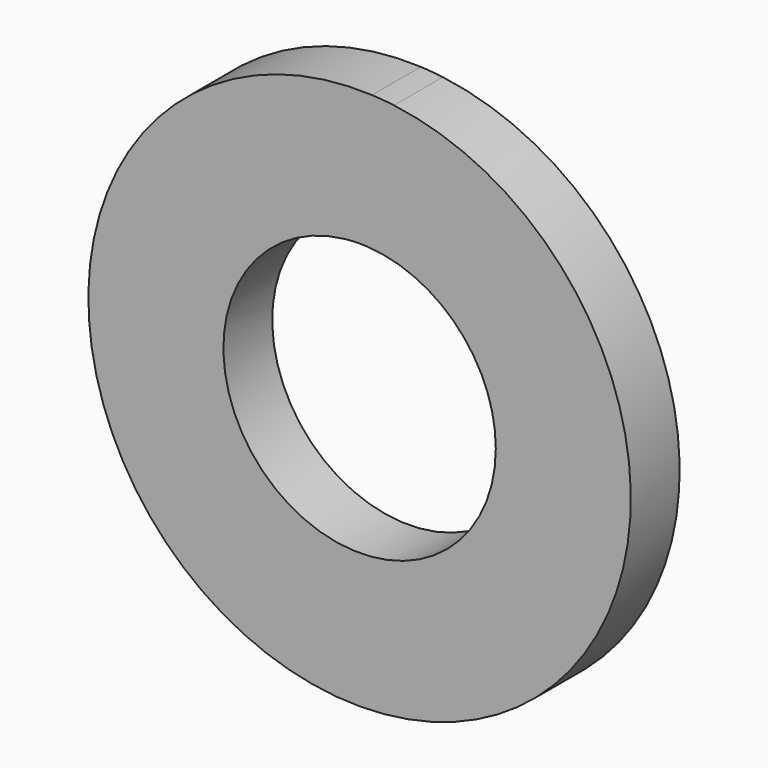
from build123d import *

# Parameters (mm, degrees)
F1_DEPTH = 15.494


# Not quite as in the source:
# - the program builds the solid bodies; features that only make, move or delete a surface that nothing else refers to are left out


with BuildPart() as f1:
    # F0 (on Front) → F1 (new body)
    with BuildSketch(Plane.XZ):
        with BuildLine():
            Line((1.9883703665, 34.5010177122), (8.7319990578, 68.2588214835))
            ThreePointArc((8.7319990578, 68.2588214835), (5.9467168888, 68.5576478309), (3.1515805748, 68.742869141))
            Line((3.1515805748, 68.742869141), (-3.7173636083, 34.3577509115))
            ThreePointArc((-3.7173636083, 34.3577509115), (-0.867459366, 34.5473783975), (1.9883703665, 34.5010177122))
        make_face()
        with BuildLine():
            ThreePointArc((3.1515805748, 68.742869141), (-49.7613844804, -47.5322956783), (68.8150747864, 0))
            ThreePointArc((68.8150747864, 0), (51.6546594513, 45.4676882503), (8.7319990578, 68.2588214835))
            Line((8.7319990578, 68.2588214835), (1.9883703665, 34.5010177122))
            ThreePointArc((1.9883703665, 34.5010177122), (25.1295490861, 23.7229762598), (34.5582673161, 0))
            ThreePointArc((34.5582673161, 0), (-23.0847156643, -25.717109919), (-3.7173636083, 34.3577509115))
            Line((-3.7173636083, 34.3577509115), (3.1515805748, 68.742869141))
        make_face()
    extrude(amount=F1_DEPTH)


solid = f1.part
